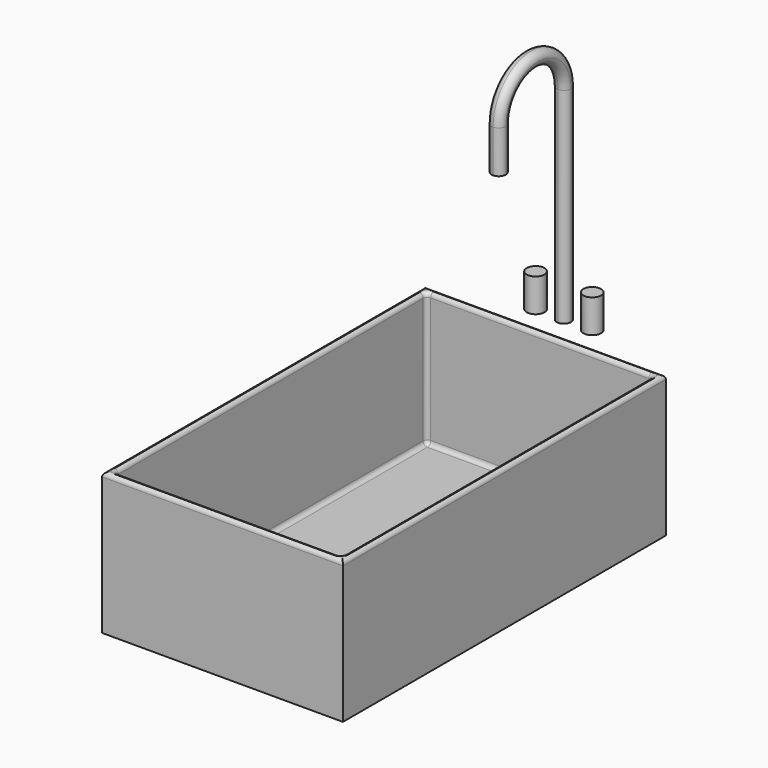
from build123d import *

# Parameters (mm, degrees)
F0_W         = 340
F0_H         = 570
F0_W_2       = 320
F0_H_2       = 550
F1_DEPTH     = 200
F2_W         = 340
F2_H         = 10.8207641169
F3_DEPTH     = 570
F4_T1_DEPTH  = 538
F4_T3_DEPTH  = 308
F4_T5_DEPTH  = 183.1792358831
F4_S9_W      = 6.12
F4_S9_H      = 6.12
F4_T10_DEPTH = 6.12
F4_S15_W     = 6.12
F4_S15_H     = 6.12
F4_T16_DEPTH = 6.12
F4_S21_W     = 6.12
F4_S21_H     = 6.12
F4_T22_DEPTH = 6.12
F4_S27_W     = 6.12
F4_S27_H     = 6.12
F4_T28_DEPTH = 6.12
F4_T31_DEPTH = 600
F4_T33_DEPTH = 370
F4_T35_DEPTH = 538
F4_T37_DEPTH = 308
F4_T40_ANGLE = 90
F4_T42_ANGLE = 90
F4_T44_ANGLE = 90
F4_T46_ANGLE = 90
F5_R         = 14.5871340725
F6_DEPTH     = 3
F12_R        = 12.5
F13_DEPTH    = 47


# Not quite as in the source:
# - a fillet or chamfer that OpenCascade refuses, or shapes differently, is made with other operations: its cross-section is extruded or revolved along the edge and cut away or added


with BuildPart() as f1:
    # F0 (on Top) → F1 (new body)
    with BuildSketch(Plane.XY):
        with Locations((152.4177306145, 254.675924629)):
            Rectangle(F0_W, F0_H)
        with Locations((152.4177306145, 254.675924629)):
            Rectangle(F0_W_2, F0_H_2, mode=Mode.SUBTRACT)
    extrude(amount=F1_DEPTH)

    # F2 (on face) → F3 (join, through all)
    with BuildSketch(Plane.XZ.offset(30.324075371)):
        with Locations((152.4177306145, 5.4103820585)):
            Rectangle(F2_W, F2_H)
    extrude(amount=-F3_DEPTH)

    # F4: fillet of radius 6 on 16 edges, made by hand

    # F4_s2 → F4_t1 (join)
    with BuildSketch(Plane.XZ.offset(-523.675924629)):
        with BuildLine():
            ThreePointArc((-1.5822693855, 10.8207641169), (-5.8249100726, 12.5781234298), (-7.5822693855, 16.8207641169))
            Line((-7.5822693855, 16.8207641169), (-7.7022693855, 16.8207641169))
            Line((-7.7022693855, 16.8207641169), (-7.7022693855, 10.7007641169))
            Line((-7.7022693855, 10.7007641169), (-1.5822693855, 10.7007641169))
            Line((-1.5822693855, 10.7007641169), (-1.5822693855, 10.8207641169))
        make_face()
        with BuildLine():
            ThreePointArc((306.4177306145, 10.8207641169), (310.6603713017, 12.5781234298), (312.4177306145, 16.8207641169))
            Line((312.4177306145, 16.8207641169), (312.5377306145, 16.8207641169))
            Line((312.5377306145, 16.8207641169), (312.5377306145, 10.7007641169))
            Line((312.5377306145, 10.7007641169), (306.4177306145, 10.7007641169))
            Line((306.4177306145, 10.7007641169), (306.4177306145, 10.8207641169))
        make_face()
    extrude(amount=F4_T1_DEPTH)

    # F4_s4 → F4_t3 (join)
    with BuildSketch(Plane.YZ.offset(-1.5822693855)):
        with BuildLine():
            ThreePointArc((523.675924629, 10.8207641169), (527.9185653161, 12.5781234298), (529.675924629, 16.8207641169))
            Line((529.675924629, 16.8207641169), (529.795924629, 16.8207641169))
            Line((529.795924629, 16.8207641169), (529.795924629, 10.7007641169))
            Line((529.795924629, 10.7007641169), (523.675924629, 10.7007641169))
            Line((523.675924629, 10.7007641169), (523.675924629, 10.8207641169))
        make_face()
        with BuildLine():
            ThreePointArc((-20.324075371, 16.8207641169), (-18.5667160581, 12.5781234298), (-14.324075371, 10.8207641169))
            Line((-14.324075371, 10.8207641169), (-14.324075371, 10.7007641169))
            Line((-14.324075371, 10.7007641169), (-20.444075371, 10.7007641169))
            Line((-20.444075371, 10.7007641169), (-20.444075371, 16.8207641169))
            Line((-20.444075371, 16.8207641169), (-20.324075371, 16.8207641169))
        make_face()
    extrude(amount=F4_T3_DEPTH)

    # F4_s6 → F4_t5 (join)
    with BuildSketch(Plane.XY.offset(16.8207641169)):
        with BuildLine():
            ThreePointArc((312.4177306145, 523.675924629), (310.6603713017, 527.9185653161), (306.4177306145, 529.675924629))
            Line((306.4177306145, 529.675924629), (306.4177306145, 529.795924629))
            Line((306.4177306145, 529.795924629), (312.5377306145, 529.795924629))
            Line((312.5377306145, 529.795924629), (312.5377306145, 523.675924629))
            Line((312.5377306145, 523.675924629), (312.4177306145, 523.675924629))
        make_face()
        with BuildLine():
            ThreePointArc((-1.5822693855, 529.675924629), (-5.8249100726, 527.9185653161), (-7.5822693855, 523.675924629))
            Line((-7.5822693855, 523.675924629), (-7.7022693855, 523.675924629))
            Line((-7.7022693855, 523.675924629), (-7.7022693855, 529.795924629))
            Line((-7.7022693855, 529.795924629), (-1.5822693855, 529.795924629))
            Line((-1.5822693855, 529.795924629), (-1.5822693855, 529.675924629))
        make_face()
        with BuildLine():
            ThreePointArc((-1.5822693855, -20.324075371), (-5.8249100726, -18.5667160581), (-7.5822693855, -14.324075371))
            Line((-7.5822693855, -14.324075371), (-7.7022693855, -14.324075371))
            Line((-7.7022693855, -14.324075371), (-7.7022693855, -20.444075371))
            Line((-7.7022693855, -20.444075371), (-1.5822693855, -20.444075371))
            Line((-1.5822693855, -20.444075371), (-1.5822693855, -20.324075371))
        make_face()
        with BuildLine():
            ThreePointArc((306.4177306145, -20.324075371), (310.6603713017, -18.5667160581), (312.4177306145, -14.324075371))
            Line((312.4177306145, -14.324075371), (312.5377306145, -14.324075371))
            Line((312.5377306145, -14.324075371), (312.5377306145, -20.444075371))
            Line((312.5377306145, -20.444075371), (306.4177306145, -20.444075371))
            Line((306.4177306145, -20.444075371), (306.4177306145, -20.324075371))
        make_face()
    extrude(amount=F4_T5_DEPTH)


with BuildPart() as f4_tool8:
    # F4_s9 → F4_t10 (new body)
    with BuildSketch(Plane.YZ.offset(-1.5822693855)):
        with Locations((-17.384075371, 13.7607641169)):
            Rectangle(F4_S9_W, F4_S9_H)
    extrude(amount=-F4_T10_DEPTH)

    # F4_s11 → F4_t12 (revolve, cut)
    with BuildSketch(Plane(origin=(-1.5822693855, -14.324075371, 16.8207641169), x_dir=(0, 0.7071067812, 0.7071067812), z_dir=(0, -0.7071067812, 0.7071067812))):
        with BuildLine():
            ThreePointArc((0, -6), (6, 0), (0, 6))
            Line((0, 6), (0, -6))
        make_face()
    revolve(axis=Axis((-1.5822693855, -14.324075371, 16.8207641169), (-1, 0, 0)), mode=Mode.SUBTRACT)


with BuildPart() as f1_1:
    add(f1.part)

    # F4_t7: union F4_tool8
    add(f4_tool8.part)


with BuildPart() as f4_tool14:
    # F4_s15 → F4_t16 (new body)
    with BuildSketch(Plane.YZ.offset(-1.5822693855)):
        with Locations((526.735924629, 13.7607641169)):
            Rectangle(F4_S15_W, F4_S15_H)
    extrude(amount=-F4_T16_DEPTH)

    # F4_s17 → F4_t18 (revolve, cut)
    with BuildSketch(Plane(origin=(-1.5822693855, 523.675924629, 16.8207641169), x_dir=(0, -0.7071067812, 0.7071067812), z_dir=(0, -0.7071067812, -0.7071067812))):
        with BuildLine():
            ThreePointArc((0, -6), (6, 0), (0, 6))
            Line((0, 6), (0, -6))
        make_face()
    revolve(axis=Axis((-1.5822693855, 523.675924629, 16.8207641169), (-1, 0, 0)), mode=Mode.SUBTRACT)


with BuildPart() as f1_2:
    add(f1_1.part)

    # F4_t13: union F4_tool14
    add(f4_tool14.part)


with BuildPart() as f4_tool20:
    # F4_s21 → F4_t22 (new body)
    with BuildSketch(Plane.XY.offset(16.8207641169)):
        with Locations((309.4777306145, 526.735924629)):
            Rectangle(F4_S21_W, F4_S21_H)
    extrude(amount=-F4_T22_DEPTH)

    # F4_s23 → F4_t24 (revolve, cut)
    with BuildSketch(Plane(origin=(306.4177306145, 523.675924629, 16.8207641169), x_dir=(-0.7071067812, -0.7071067812, 0), z_dir=(0.7071067812, -0.7071067812, 0))):
        with BuildLine():
            ThreePointArc((0, -6), (6, 0), (0, 6))
            Line((0, 6), (0, -6))
        make_face()
    revolve(axis=Axis((306.4177306145, 523.675924629, 16.8207641169), (0, 0, -1)), mode=Mode.SUBTRACT)


with BuildPart() as f1_3:
    add(f1_2.part)

    # F4_t19: union F4_tool20
    add(f4_tool20.part)


with BuildPart() as f4_tool26:
    # F4_s27 → F4_t28 (new body)
    with BuildSketch(Plane.XZ.offset(14.324075371)):
        with Locations((309.4777306145, 13.7607641169)):
            Rectangle(F4_S27_W, F4_S27_H)
    extrude(amount=F4_T28_DEPTH)

    # F4_s29 → F4_t30 (revolve, cut)
    with BuildSketch(Plane(origin=(306.4177306145, -14.324075371, 16.8207641169), x_dir=(-0.7071067812, 0, 0.7071067812), z_dir=(0.7071067812, 0, 0.7071067812))):
        with BuildLine():
            ThreePointArc((0, -6), (6, 0), (0, 6))
            Line((0, 6), (0, -6))
        make_face()
    revolve(axis=Axis((306.4177306145, -14.324075371, 16.8207641169), (0, -1, 0)), mode=Mode.SUBTRACT)


with BuildPart() as f1_4:
    add(f1_3.part)

    # F4_t25: union F4_tool26
    add(f4_tool26.part)

    # F4_s32 → F4_t31 (cut)
    with BuildSketch(Plane.XZ.offset(-554.675924629)):
        with BuildLine():
            ThreePointArc((-17.5822693855, 194), (-15.8249100726, 198.2426406871), (-11.5822693855, 200))
            Line((-11.5822693855, 200), (-11.5822693855, 200.12))
            Line((-11.5822693855, 200.12), (-17.7022693855, 200.12))
            Line((-17.7022693855, 200.12), (-17.7022693855, 194))
            Line((-17.7022693855, 194), (-17.5822693855, 194))
        make_face()
        with BuildLine():
            ThreePointArc((316.4177306145, 200), (320.6603713017, 198.2426406871), (322.4177306145, 194))
            Line((322.4177306145, 194), (322.5377306145, 194))
            Line((322.5377306145, 194), (322.5377306145, 200.12))
            Line((322.5377306145, 200.12), (316.4177306145, 200.12))
            Line((316.4177306145, 200.12), (316.4177306145, 200))
        make_face()
    extrude(amount=F4_T31_DEPTH, mode=Mode.SUBTRACT)

    # F4_s34 → F4_t33 (cut)
    with BuildSketch(Plane.YZ.offset(-32.5822693855)):
        with BuildLine():
            ThreePointArc((-24.324075371, 200), (-28.5667160581, 198.2426406871), (-30.324075371, 194))
            Line((-30.324075371, 194), (-30.444075371, 194))
            Line((-30.444075371, 194), (-30.444075371, 200.12))
            Line((-30.444075371, 200.12), (-24.324075371, 200.12))
            Line((-24.324075371, 200.12), (-24.324075371, 200))
        make_face()
        with BuildLine():
            ThreePointArc((539.675924629, 194), (537.9185653161, 198.2426406871), (533.675924629, 200))
            Line((533.675924629, 200), (533.675924629, 200.12))
            Line((533.675924629, 200.12), (539.795924629, 200.12))
            Line((539.795924629, 200.12), (539.795924629, 194))
            Line((539.795924629, 194), (539.675924629, 194))
        make_face()
    extrude(amount=F4_T33_DEPTH, mode=Mode.SUBTRACT)

    # F4_s36 → F4_t35 (cut)
    with BuildSketch(Plane.XZ.offset(-523.675924629)):
        with BuildLine():
            ThreePointArc((-13.5822693855, 200), (-9.3396286983, 198.2426406871), (-7.5822693855, 194))
            Line((-7.5822693855, 194), (-7.4622693855, 194))
            Line((-7.4622693855, 194), (-7.4622693855, 200.12))
            Line((-7.4622693855, 200.12), (-13.5822693855, 200.12))
            Line((-13.5822693855, 200.12), (-13.5822693855, 200))
        make_face()
        with BuildLine():
            ThreePointArc((318.4177306145, 200), (314.1750899274, 198.2426406871), (312.4177306145, 194))
            Line((312.4177306145, 194), (312.2977306145, 194))
            Line((312.2977306145, 194), (312.2977306145, 200.12))
            Line((312.2977306145, 200.12), (318.4177306145, 200.12))
            Line((318.4177306145, 200.12), (318.4177306145, 200))
        make_face()
    extrude(amount=F4_T35_DEPTH, mode=Mode.SUBTRACT)

    # F4_s38 → F4_t37 (cut)
    with BuildSketch(Plane.YZ.offset(-1.5822693855)):
        with BuildLine():
            ThreePointArc((535.675924629, 200), (531.4332839419, 198.2426406871), (529.675924629, 194))
            Line((529.675924629, 194), (529.555924629, 194))
            Line((529.555924629, 194), (529.555924629, 200.12))
            Line((529.555924629, 200.12), (535.675924629, 200.12))
            Line((535.675924629, 200.12), (535.675924629, 200))
        make_face()
        with BuildLine():
            ThreePointArc((-26.324075371, 200), (-22.0814346839, 198.2426406871), (-20.324075371, 194))
            Line((-20.324075371, 194), (-20.204075371, 194))
            Line((-20.204075371, 194), (-20.204075371, 200.12))
            Line((-20.204075371, 200.12), (-26.324075371, 200.12))
            Line((-26.324075371, 200.12), (-26.324075371, 200))
        make_face()
    extrude(amount=F4_T37_DEPTH, mode=Mode.SUBTRACT)

    # F4_s39 → F4_t40 (revolve, cut)
    with BuildSketch(Plane.YZ.offset(306.4177306145)):
        with BuildLine():
            ThreePointArc((-26.324075371, 200), (-22.0814346839, 198.2426406871), (-20.324075371, 194))
            Line((-20.324075371, 194), (-20.204075371, 194))
            Line((-20.204075371, 194), (-20.204075371, 200.12))
            Line((-20.204075371, 200.12), (-26.324075371, 200.12))
            Line((-26.324075371, 200.12), (-26.324075371, 200))
        make_face()
    revolve(axis=Axis((306.4177306145, -14.324075371, 200), (0, 0, 1)), revolution_arc=F4_T40_ANGLE, mode=Mode.SUBTRACT)

    # F4_s41 → F4_t42 (revolve, cut)
    with BuildSketch(Plane.YZ.offset(-1.5822693855)):
        with BuildLine():
            ThreePointArc((-26.324075371, 200), (-22.0814346839, 198.2426406871), (-20.324075371, 194))
            Line((-20.324075371, 194), (-20.204075371, 194))
            Line((-20.204075371, 194), (-20.204075371, 200.12))
            Line((-20.204075371, 200.12), (-26.324075371, 200.12))
            Line((-26.324075371, 200.12), (-26.324075371, 200))
        make_face()
    revolve(axis=Axis((-1.5822693855, -14.324075371, 200), (0, 0, -1)), revolution_arc=F4_T42_ANGLE, mode=Mode.SUBTRACT)

    # F4_s43 → F4_t44 (revolve, cut)
    with BuildSketch(Plane.XZ.offset(-523.675924629)):
        with BuildLine():
            ThreePointArc((318.4177306145, 200), (314.1750899274, 198.2426406871), (312.4177306145, 194))
            Line((312.4177306145, 194), (312.2977306145, 194))
            Line((312.2977306145, 194), (312.2977306145, 200.12))
            Line((312.2977306145, 200.12), (318.4177306145, 200.12))
            Line((318.4177306145, 200.12), (318.4177306145, 200))
        make_face()
    revolve(axis=Axis((306.4177306145, 523.675924629, 200), (0, 0, 1)), revolution_arc=F4_T44_ANGLE, mode=Mode.SUBTRACT)

    # F4_s45 → F4_t46 (revolve, cut)
    with BuildSketch(Plane.YZ.offset(-1.5822693855)):
        with BuildLine():
            ThreePointArc((535.675924629, 200), (531.4332839419, 198.2426406871), (529.675924629, 194))
            Line((529.675924629, 194), (529.555924629, 194))
            Line((529.555924629, 194), (529.555924629, 200.12))
            Line((529.555924629, 200.12), (535.675924629, 200.12))
            Line((535.675924629, 200.12), (535.675924629, 200))
        make_face()
    revolve(axis=Axis((-1.5822693855, 523.675924629, 200), (0, 0, 1)), revolution_arc=F4_T46_ANGLE, mode=Mode.SUBTRACT)

    # F5 (on face) → F6 (cut)
    with BuildSketch(Plane.XY.offset(10.8207641169)):
        with Locations((152.4177306145, 467.7632451057)):
            Circle(F5_R)
    extrude(amount=-F6_DEPTH, mode=Mode.SUBTRACT)


with BuildPart() as f11:
    # F11: sweep along a path in F10
    with BuildLine(Plane.YZ.offset(152.4177306145)) as f11_path:
        Line((572.175924629, 200), (572.175924629, 430))
        Line((572.175924629, 430), (572.175924629, 490))
        ThreePointArc((572.175924629, 490), (514.681654498, 547.494270131), (457.187384367, 490))
        Line((457.187384367, 490), (457.187384367, 430))
    # F8 (on offset) → F11 (sweep)
    with BuildSketch(Plane.XY.offset(200)):
        with BuildLine():
            ThreePointArc((152.4177306145, 582.175924629), (142.4177306145, 572.175924629), (152.4177306145, 562.175924629))
            Line((152.4177306145, 562.175924629), (152.4177306145, 582.175924629))
        make_face()
        with BuildLine():
            Line((152.4177306145, 582.175924629), (152.4177306145, 562.175924629))
            ThreePointArc((152.4177306145, 562.175924629), (159.4887984264, 565.1048568171), (162.4177306145, 572.175924629))
            ThreePointArc((162.4177306145, 572.175924629), (159.4887984264, 579.2469924408), (152.4177306145, 582.175924629))
        make_face()
    sweep(path=f11_path.line)


with BuildPart() as f13:
    # F12 (on offset) → F13 (new body)
    with BuildSketch(Plane.XY.offset(200)):
        with Locations((112.4177306145, 572.175924629)):
            Circle(F12_R)
    extrude(amount=F13_DEPTH)


with BuildPart() as f13b:
    # F12 (on offset) → F13, piece 2 (new body)
    with BuildSketch(Plane.XY.offset(200)):
        with Locations((192.4177306145, 572.175924629)):
            Circle(F12_R)
    extrude(amount=F13_DEPTH)


solid = Compound([f1_4.part, f11.part, f13.part, f13b.part])
